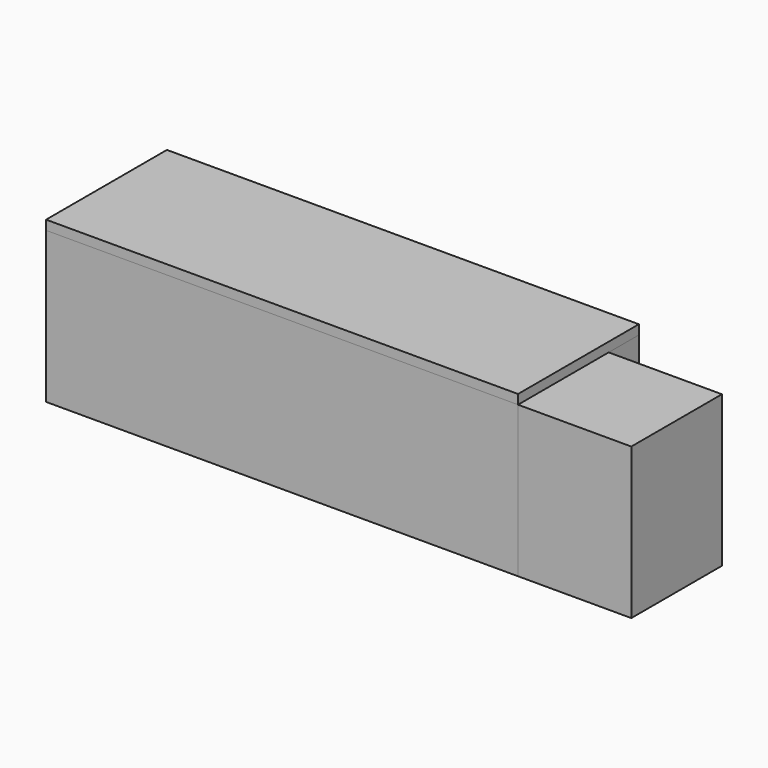
from build123d import *

# Parameters (mm, degrees)
F0_W     = 900
F0_H     = 80
F1_DEPTH = 800
F2_W     = 2500
F2_H     = 50
F3_DEPTH = 800
F0_W_2   = 600
F0_H_2   = 600
F4_DEPTH = 800


with BuildPart() as f1:
    # F0 (on Top) → F1 (new body)
    with BuildSketch(Plane.XY):
        Polygon((-450, 400), (-1250, 400), (-1250, -400), (-450, -400), (-450, -320), (-1170, -320), (-1170, 320), (-450, 320), align=None)
        with Locations((0, 360)):
            Rectangle(F0_W, F0_H)
        Polygon((1250, 400), (450, 400), (450, 320), (1170, 320), (1170, -320), (450, -320), (450, -400), (1250, -400), (1250, 200), align=None)
        with Locations((0, -360)):
            Rectangle(F0_W, F0_H)
    extrude(amount=-F1_DEPTH)


with BuildPart() as f3:
    # F2 (on face) → F3 (new body)
    with BuildSketch(Plane.XZ.offset(400)):
        with Locations((0, 25)):
            Rectangle(F2_W, F2_H)
    extrude(amount=-F3_DEPTH)


with BuildPart() as f4:
    # F0 (on Top) → F4 (new body)
    with BuildSketch(Plane.XY):
        with Locations((1550, -100)):
            Rectangle(F0_W_2, F0_H_2)
    extrude(amount=-F4_DEPTH)


solid = Compound([f1.part, f3.part, f4.part])
